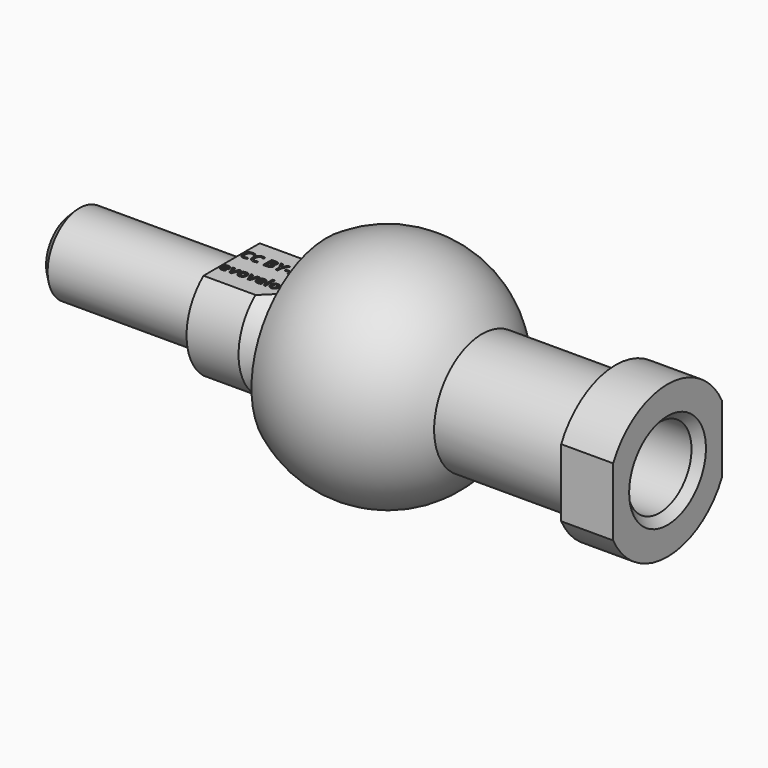
from build123d import *

# Parameters (mm, degrees)
F4_DEPTH      = 6.5
F5_D          = 10
F5_DEPTH      = 18
F5_TIP        = 3.0043030951
F6_D          = 8
F6_DEPTH      = 4
F6_START      = 18.6008606
F6_TIP        = 2.4034424761
F7_D          = 2
F9_DEPTH      = 9.3445980781
F10_SIZE      = 1
F10_2_SIZE    = 1
F11_TEXT_SIZE = 1.9184829842
F12_DEPTH     = 0.2


# Not quite as in the source:
# - Text() gives the source's letters only with a copy of the font that has no kerning and outlines rounded to 1/6400 em; it was checked with that copy


with BuildPart() as f1:
    # F0 (on Top) → F1 (revolve)
    with BuildSketch(Plane.XY):
        with BuildLine():
            ThreePointArc((-7.6243874277, 7.2193293561), (3.8854814379, 9.7546416641), (10.5, 0))
            Line((10.5, 0), (35, 0))
            Line((35, 0), (35, 9.5))
            Line((35, 9.5), (28.5, 9.5))
            Line((28.5, 9.5), (28.5, 7.5))
            Line((28.5, 7.5), (11.8215904175, 7.5))
            ThreePointArc((11.8215904175, 7.5), (2.9836623642, 13.6783682834), (-7.6243874277, 11.7417509917))
            Line((-7.6243874277, 11.7417509917), (-7.6243874277, 7.2193293561))
        make_face()
    revolve(axis=Axis((5.2878996746, 0, 0), (1, 0, 0)))

    # F3 (on face) → F4 (cut, through all)
    with BuildSketch(Plane.YZ.offset(35)):
        with BuildLine():
            ThreePointArc((9.5, 0), (9.2466210045, 2.1794494718), (8.5, 4.2426406871))
            Line((8.5, 4.2426406871), (8.5, -4.2426406871))
            ThreePointArc((8.5, -4.2426406871), (9.2466210045, -2.1794494718), (9.5, 0))
        make_face()
        with BuildLine():
            Line((-8.5, -4.2426406871), (-8.5, 4.2426406871))
            ThreePointArc((-8.5, 4.2426406871), (-9.5, 0), (-8.5, -4.2426406871))
        make_face()
    extrude(amount=-F4_DEPTH, mode=Mode.SUBTRACT)

    # F5
    with Locations(Plane.YZ.offset(35)):
        with Locations((0, 0)):
            Hole(F5_D / 2, depth=F5_DEPTH)
            with Locations((0, 0, -(F5_DEPTH + F5_TIP / 2))):  # 118° drill point
                Cone(0, F5_D / 2, F5_TIP, mode=Mode.SUBTRACT)

    # F6
    # its depths count from where the whole tool has entered the part; down to there all is cleared
    with Locations(Plane.YZ.offset(35)):
        with Locations((0, 0)):
            Hole(F6_D / 2, depth=F6_START)
    with Locations(Plane.YZ.offset(35).offset(-F6_START)):
        with Locations((0, 0)):
            Hole(F6_D / 2, depth=F6_DEPTH)
            with Locations((0, 0, -(F6_DEPTH + F6_TIP / 2))):  # 118° drill point
                Cone(0, F6_D / 2, F6_TIP, mode=Mode.SUBTRACT)

    # F7 (through all)
    with Locations(Plane.YZ.offset(35)):
        with Locations((0, 0)):
            Hole(F7_D / 2)

    # F10#2
    f10_2_edges = [f1.edges().sort_by_distance(p)[0] for p in [
        (35, -5, 0),
    ]]
    chamfer(f10_2_edges, length=F10_2_SIZE)


with BuildPart() as f2:
    # F0 (on Top) → F2 (revolve)
    with BuildSketch(Plane.XY):
        with BuildLine():
            Line((-39.5, 0), (10.5, 0))
            ThreePointArc((10.5, 0), (3.8854814379, 9.7546416641), (-7.6243874277, 7.2193293561))
            ThreePointArc((-7.6243874277, 7.2193293561), (-8.5014713076, 6.1623847337), (-9.2330926563, 5))
            Line((-9.2330926563, 5), (-13, 7.039894694))
            Line((-13, 7.039894694), (-19.5, 7.039894694))
            Line((-19.5, 7.039894694), (-19.5, 5))
            Line((-19.5, 5), (-39.5, 5))
            Line((-39.5, 5), (-39.5, 0))
        make_face()
    revolve(axis=Axis((5.2878996746, 0, 0), (1, 0, 0)))

    # F8 (on face) → F9 (cut, through all)
    with BuildSketch(Plane(origin=(-19.5, 0, 0), x_dir=(0, -1, 0), z_dir=(-1, 0, 0))):
        with BuildLine():
            ThreePointArc((4.3943278555, 5.5), (0, 7.039894694), (-4.3943278555, 5.5))
            Line((-4.3943278555, 5.5), (4.3943278555, 5.5))
        make_face()
        with BuildLine():
            Line((4.3943278555, -5.5), (-4.3943278555, -5.5))
            ThreePointArc((-4.3943278555, -5.5), (0, -7.039894694), (4.3943278555, -5.5))
        make_face()
    extrude(amount=-F9_DEPTH, mode=Mode.SUBTRACT)

    # F10
    f10_edges = [f2.edges().sort_by_distance(p)[0] for p in [
        (-39.5, -5, 0),
    ]]
    chamfer(f10_edges, length=F10_SIZE)

    # F11 (on face) → F12 (cut)
    with BuildSketch(Plane.XY.offset(5.5)):
        with Locations((-19.5, 1.0072681858)):
            Text('CC BY-SA', F11_TEXT_SIZE, font='Open Sans', font_style=FontStyle.BOLD, text_align=(TextAlign.LEFT, TextAlign.BOTTOM))
        with Locations((-19.5, -2.2833068388)):
            Text('evovelo', F11_TEXT_SIZE, font='Open Sans', font_style=FontStyle.BOLD, text_align=(TextAlign.LEFT, TextAlign.BOTTOM))
    extrude(amount=-F12_DEPTH, mode=Mode.SUBTRACT)


solid = Compound([f1.part, f2.part])
